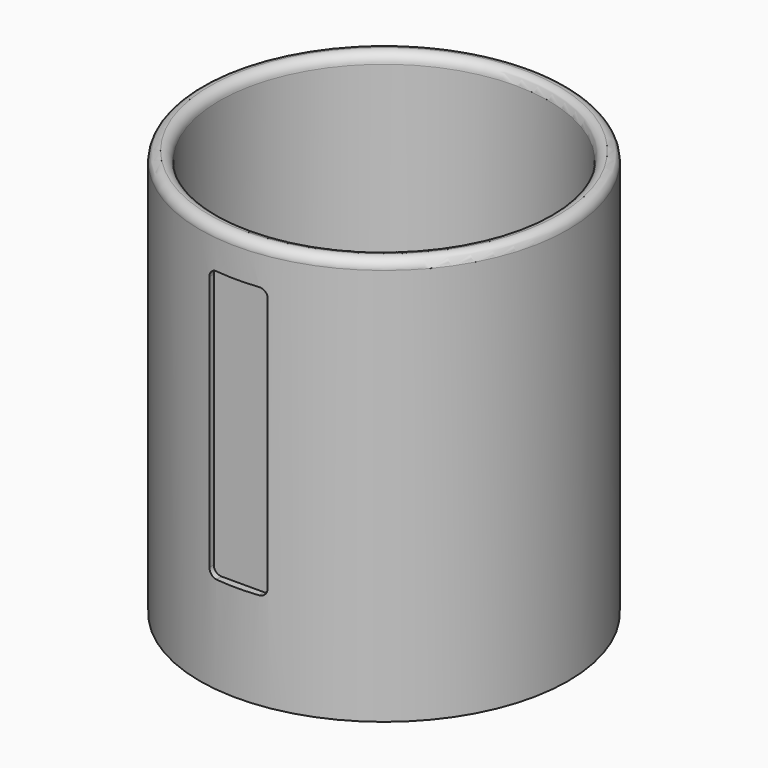
from build123d import *

# Parameters (mm, degrees)
F0_R     = 47.5
F1_DEPTH = 5
F2_R     = 47.5
F2_R_2   = 42.5
F3_DEPTH = 100
F6_DEPTH = 2
F8_R     = 2.49999


# Not quite as in the source:
# - a fillet or chamfer is up to 0.001 mm smaller than in the source, because OpenCascade refuses the exact size


with BuildPart() as f1:
    # F0 (on Top) → F1 (new body)
    with BuildSketch(Plane.XY):
        Circle(F0_R)
    extrude(amount=F1_DEPTH)

    # F2 (on face) → F3 (join)
    with BuildSketch(Plane.XY.offset(5)):
        Circle(F2_R)
        Circle(F2_R_2, mode=Mode.SUBTRACT)
    extrude(amount=F3_DEPTH)

    # F5 (on offset) → F6 (cut)
    with BuildSketch(Plane.XZ.offset(47.5)):
        with BuildLine():
            ThreePointArc((7.5, 93), (6.9142135624, 94.4142135624), (5.5, 95))
            Line((5.5, 95), (-5.5, 95))
            ThreePointArc((-5.5, 95), (-6.9142135624, 94.4142135624), (-7.5, 93))
            Line((-7.5, 93), (-7.5, 27))
            ThreePointArc((-7.5, 27), (-6.9142135624, 25.5857864376), (-5.5, 25))
            Line((-5.5, 25), (5.5, 25))
            ThreePointArc((5.5, 25), (6.9142135624, 25.5857864376), (7.5, 27))
            Line((7.5, 27), (7.5, 93))
        make_face()
    extrude(amount=-F6_DEPTH, mode=Mode.SUBTRACT)

    # F8 (radius 2.5 in the source; OpenCascade refuses exactly that, so slightly less here)
    f8_edges = [f1.edges().sort_by_distance(p)[0] for p in [
        (-47.5, 0, 105),
        (-42.5, 0, 105),
    ]]
    fillet(f8_edges, radius=F8_R)


solid = f1.part
